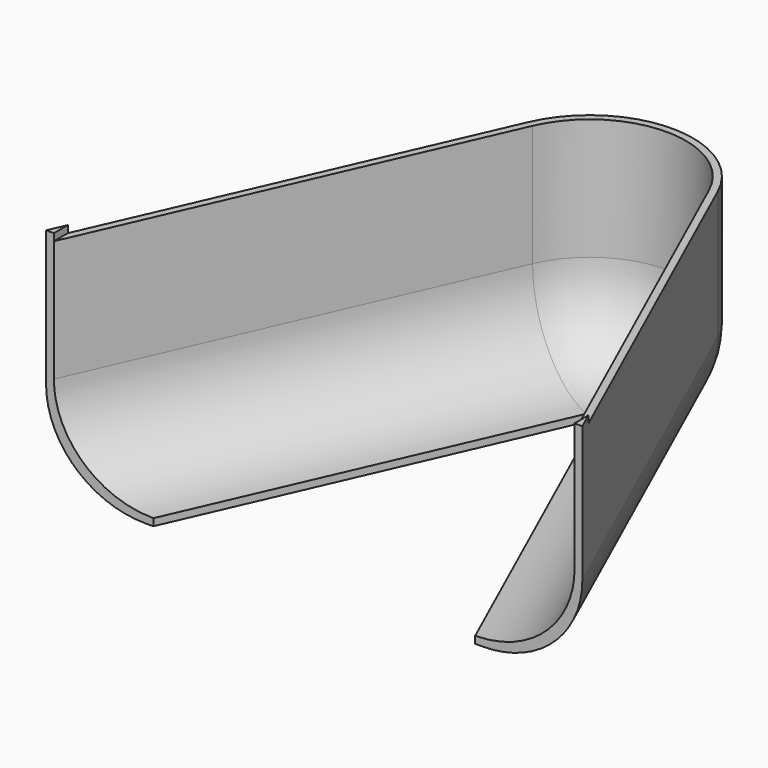
from build123d import *

# Parameters (mm, degrees)
F1_DEPTH = 63.5
F2_T     = -2
F3_R     = 25.4
F4_ANGLE = 180
F5_ANGLE = -48
F6_W     = 145.6223272032
F6_H     = 2
F7_DEPTH = 127
F8_DEPTH = 25.4


# Not quite as in the source:
# - a feature names something its author has since deleted; it is built from what else it names


with BuildPart() as f1:
    # F0 (on Top) → F1 (new body)
    with BuildSketch(Plane.XY):
        with BuildLine():
            Line((-10.2850095064, 143.0450051312), (-58.2692639971, 33.9835022184))
            Line((-58.2692639971, 33.9835022184), (91.7307360029, 34.4206405823))
            Line((91.7307360029, 34.4206405823), (42.7254554371, 143.2713651338))
            ThreePointArc((42.7254554371, 143.2713651338), (44.5808039736, 137.7049772305), (45.2782310553, 131.8791221047))
            Line((45.2782310553, 131.8791221047), (45.4024820726, 131.3612216192))
            Line((45.4024820726, 131.3612216192), (45.2828539684, 131.3612216192))
            ThreePointArc((45.2828539684, 131.3612216192), (16.2705971829, 102.3489648337), (-12.7416596027, 131.3612216192))
            ThreePointArc((-12.7416596027, 131.3612216192), (-12.1208550885, 137.3308515669), (-10.2850095064, 143.0450051312))
        make_face()
        with BuildLine():
            ThreePointArc((42.7254554371, 143.2713651338), (16.1467130657, 160.3732139071), (-10.2850095064, 143.0450051312))
            ThreePointArc((-10.2850095064, 143.0450051312), (-12.1208550885, 137.3308515669), (-12.7416596027, 131.3612216192))
            Line((-12.7416596027, 131.3612216192), (45.2828539684, 131.3612216192))
            ThreePointArc((45.2828539684, 131.3612216192), (45.2816982171, 131.6201821781), (45.2782310553, 131.8791221047))
            ThreePointArc((45.2782310553, 131.8791221047), (44.5808039736, 137.7049772305), (42.7254554371, 143.2713651338))
        make_face()
        with BuildLine():
            Line((45.2828539684, 131.3612216192), (-12.7416596027, 131.3612216192))
            ThreePointArc((-12.7416596027, 131.3612216192), (16.2705971829, 102.3489648337), (45.2828539684, 131.3612216192))
        make_face()
        with BuildLine():
            Line((45.4024820726, 131.3612216192), (45.2782310553, 131.8791221047))
            ThreePointArc((45.2782310553, 131.8791221047), (45.2816982171, 131.6201821781), (45.2828539684, 131.3612216192))
            Line((45.2828539684, 131.3612216192), (45.4024820726, 131.3612216192))
        make_face()
    extrude(amount=F1_DEPTH)

    # F2
    f2_openings = [f1.faces().sort_by_distance(p)[0] for p in [
        (16.730736, 34.202071, 31.75),
    ]]
    offset(amount=F2_T, openings=f2_openings)

    # F3
    f3_edges = [f1.edges().sort_by_distance(p)[0] for p in [
        (16.146713, 160.373214, 63.5),
        (16.155253, 158.373232, 61.5),
    ]]
    fillet(f3_edges, radius=F3_R)


with BuildPart() as f1_1:
    # F4: moved
    add(f1.part.rotate(Axis((41.7381236511, 83.5918491789, 63.5), (-0.4105210981, 0.9118510997, 0)), F4_ANGLE))


with BuildPart() as f1_2:
    # F5: moved
    add(f1_1.part.rotate(Axis((45.4087001389, 13.5661687977, 95.25), (0, 0, 1)), F5_ANGLE))

    # F6 (on face) → F7 (cut)
    with BuildSketch(Plane(origin=(-0.0716524101, 13.3215442397, 0), x_dir=(0.9999855352, 0.0053786087, 0), z_dir=(0.0053786087, -0.9999855352, 0))):
        with Locations((120.4826499572, 126)):
            Rectangle(F6_W, F6_H)
    extrude(amount=-F7_DEPTH, mode=Mode.SUBTRACT)

    # F8 (cut): a face of the model
    f8_faces = [f1_2.faces().sort_by_distance(p)[0] for p in [
        (120.299637411, 47.6367123165, 65.5),
    ]]
    extrude(f8_faces, amount=-F8_DEPTH, mode=Mode.SUBTRACT)


solid = f1_2.part
